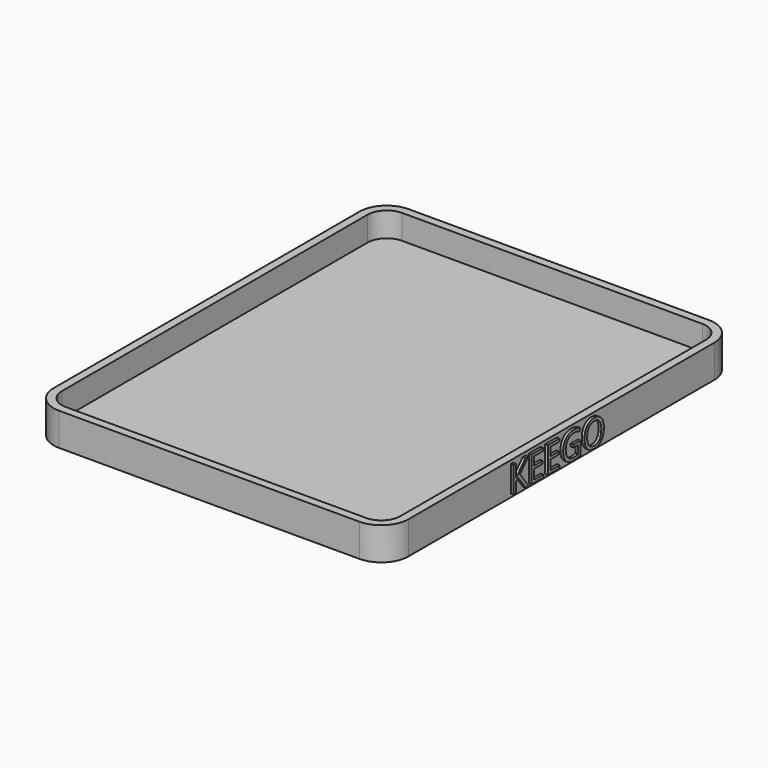
from build123d import *

# Parameters (mm, degrees)
F1_DEPTH     = 1.5
F2_DEPTH     = 6
F3_TEXT_SIZE = 6.7292013328
F4_DEPTH     = 0.5


# Not quite as in the source:
# - Text() gives the source's letters only with a copy of the font that has no kerning and outlines rounded to 1/6400 em; it was checked with that copy


with BuildPart() as f1:
    # F0 (on Top) → F1 (new body)
    with BuildSketch(Plane.XY):
        with BuildLine():
            Line((-28.0414680019, 53.8901910931), (-28.0414680019, -16.1098089069))
            ThreePointArc((-28.0414680019, -16.1098089069), (-27.0163417361, -18.5846826411), (-24.5414680019, -19.6098089069))
            Line((-24.5414680019, -19.6098089069), (30.4585319981, -19.6098089069))
            ThreePointArc((30.4585319981, -19.6098089069), (32.9334057323, -18.5846826411), (33.9585319981, -16.1098089069))
            Line((33.9585319981, -16.1098089069), (33.9585319981, 53.8901910931))
            ThreePointArc((33.9585319981, 53.8901910931), (32.9334057323, 56.3650648272), (30.4585319981, 57.3901910931))
            Line((30.4585319981, 57.3901910931), (-24.5414680019, 57.3901910931))
            ThreePointArc((-24.5414680019, 57.3901910931), (-27.0163417361, 56.3650648272), (-28.0414680019, 53.8901910931))
        make_face()
    extrude(amount=F1_DEPTH)

    # F0 (on Top) → F2 (join)
    with BuildSketch(Plane.XY):
        with BuildLine():
            ThreePointArc((-29.5414680019, -16.1098089069), (-28.0770019078, -19.6453428128), (-24.5414680019, -21.1098089069))
            Line((-24.5414680019, -21.1098089069), (30.4585319981, -21.1098089069))
            ThreePointArc((30.4585319981, -21.1098089069), (33.994065904, -19.6453428128), (35.4585319981, -16.1098089069))
            Line((35.4585319981, -16.1098089069), (35.4585319981, 53.8901910931))
            ThreePointArc((35.4585319981, 53.8901910931), (33.994065904, 57.425724999), (30.4585319981, 58.8901910931))
            Line((30.4585319981, 58.8901910931), (-24.5414680019, 58.8901910931))
            ThreePointArc((-24.5414680019, 58.8901910931), (-28.0770019078, 57.425724999), (-29.5414680019, 53.8901910931))
            Line((-29.5414680019, 53.8901910931), (-29.5414680019, -16.1098089069))
        make_face()
        with BuildLine():
            ThreePointArc((-24.5414680019, -19.6098089069), (-27.0163417361, -18.5846826411), (-28.0414680019, -16.1098089069))
            Line((-28.0414680019, -16.1098089069), (-28.0414680019, 53.8901910931))
            ThreePointArc((-28.0414680019, 53.8901910931), (-27.0163417361, 56.3650648272), (-24.5414680019, 57.3901910931))
            Line((-24.5414680019, 57.3901910931), (30.4585319981, 57.3901910931))
            ThreePointArc((30.4585319981, 57.3901910931), (32.9334057323, 56.3650648272), (33.9585319981, 53.8901910931))
            Line((33.9585319981, 53.8901910931), (33.9585319981, -16.1098089069))
            ThreePointArc((33.9585319981, -16.1098089069), (32.9334057323, -18.5846826411), (30.4585319981, -19.6098089069))
            Line((30.4585319981, -19.6098089069), (-24.5414680019, -19.6098089069))
        make_face(mode=Mode.SUBTRACT)
    extrude(amount=F2_DEPTH)

    # F3 (on face) → F4 (join)
    with BuildSketch(Plane.YZ.offset(35.4585319981)):
        with Locations((6.6344507504, 0.5806740955)):
            Text('KEEGO', F3_TEXT_SIZE, font='Open Sans', text_align=(TextAlign.LEFT, TextAlign.BOTTOM))
    extrude(amount=F4_DEPTH)


solid = f1.part
